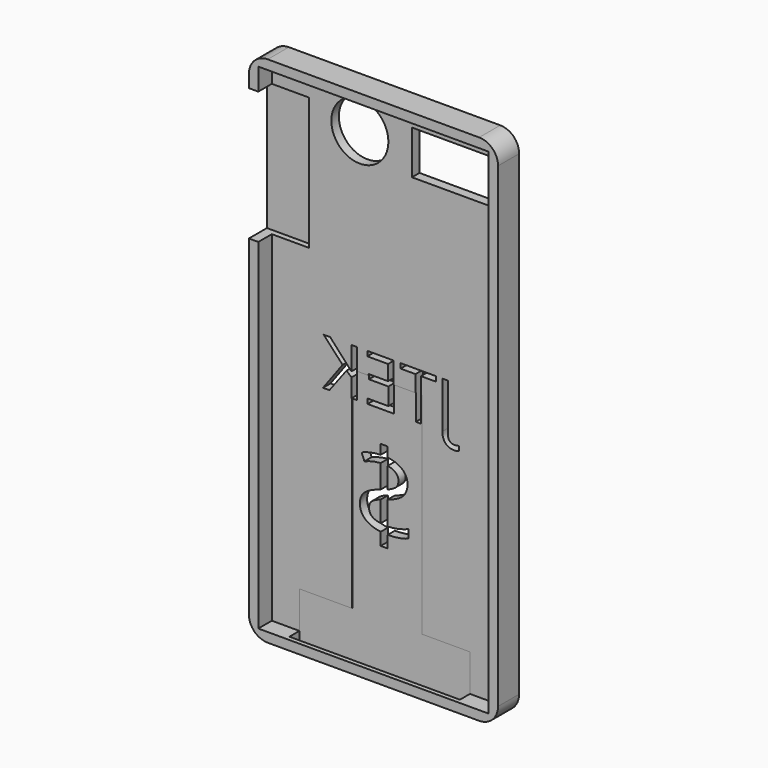
from build123d import *

# Parameters (mm, degrees)
F0_W          = 67.1
F0_H          = 138.3
F1_DEPTH      = 3.55
F2_T          = -2.54
F3_R          = 5.08
F4_R          = 5.08
F5_R          = 5.08
F6_R          = 5.08
F7_W          = 21.1026063189
F7_H          = 11.7926336825
F8_DEPTH      = 12.5
F11_W         = 18.811494112
F11_H         = 2.224416472
F12_DEPTH     = 91.3
F13_W         = 6.076481403
F13_H         = 22.8435061872
F14_DEPTH     = 12.5
F15_R         = 7.6799420763
F16_DEPTH     = 25
F18_DEPTH     = 12.5
F19_W         = 6.076481403
F19_H         = 12.7864610404
F20_DEPTH     = 12.5
F21_R         = 12.4287967825
F22_DEPTH     = 25
F23_DEPTH     = 108.6
F24_TEXT_SIZE = 17.723527142
F25_DEPTH     = 12.5
F26_TEXT_SIZE = 29.6242431634
F27_DEPTH     = 25


# Not quite as in the source:
# - a feature of the source that left no trace in its solid (it failed there, or was rolled back) is left out
# - Text() gives the source's letters only with a copy of the font that has no kerning and outlines rounded to 1/6400 em; it was checked with that copy


with BuildPart() as f1:
    # F0 (on Front) → F1 (new body, symmetric)
    with BuildSketch(Plane.XZ):
        Rectangle(F0_W, F0_H)
    extrude(amount=F1_DEPTH, both=True)

    # F2
    f2_openings = [f1.faces().sort_by_distance(p)[0] for p in [
        (0, -3.55, 0),
    ]]
    offset(amount=F2_T, openings=f2_openings)

    # F3
    f3_edges = [f1.edges().sort_by_distance(p)[0] for p in [
        (33.55, 0, 69.15),
    ]]
    fillet(f3_edges, radius=F3_R)

    # F4
    f4_edges = [f1.edges().sort_by_distance(p)[0] for p in [
        (-33.55, 0, 69.15),
    ]]
    fillet(f4_edges, radius=F4_R)

    # F5
    f5_edges = [f1.edges().sort_by_distance(p)[0] for p in [
        (-33.55, 0, -69.15),
    ]]
    fillet(f5_edges, radius=F5_R)

    # F6
    f6_edges = [f1.edges().sort_by_distance(p)[0] for p in [
        (33.55, 0, -69.15),
    ]]
    fillet(f6_edges, radius=F6_R)

    # F7 (on face) → F8 (cut, symmetric)
    with BuildSketch(Plane.XZ.offset(-1.01)):
        with Locations((17.2698632814, 56.677794084)):
            Rectangle(F7_W, F7_H)
    extrude(amount=F8_DEPTH, both=True, mode=Mode.SUBTRACT)

    # F11 (on Top) → F12 (cut)
    with BuildSketch(Plane.XY):
        Rectangle(F11_W, F11_H)
    extrude(amount=-F12_DEPTH, mode=Mode.SUBTRACT)

    # F13 (on face) → F14 (cut, symmetric)
    with BuildSketch(Plane(origin=(-33.55, 0, 0), x_dir=(0, -1, 0), z_dir=(-1, 0, 0))):
        with Locations((0.5117592985, 49.2424760014)):
            Rectangle(F13_W, F13_H)
    extrude(amount=F14_DEPTH, both=True, mode=Mode.SUBTRACT)

    # F15 (on face) → F16 (cut)
    with BuildSketch(Plane.XZ.offset(-1.01)):
        with Locations((-7.3086209595, 57.1251362562)):
            Circle(F15_R)
    extrude(amount=-F16_DEPTH, mode=Mode.SUBTRACT)

    # F17 (on face) → F18 (cut, symmetric)
    with BuildSketch(Plane(origin=(0, 0, -69.15), x_dir=(1, 0, 0), z_dir=(0, 0, -1))):
        Polygon((22.3355982453, 2.3663339671), (-23.5800333321, 2.3663339671), (-23.5800333321, -1.112208236), (-9.405747056, -1.112208236), (-9.405747056, 1.112208236), (9.405747056, 1.112208236), (9.405747056, -1.112208236), (22.3355982453, -1.112208236), align=None)
    extrude(amount=F18_DEPTH, both=True, mode=Mode.SUBTRACT)

    # F19 (on face) → F20 (cut, symmetric)
    with BuildSketch(Plane(origin=(-33.55, 0, 0), x_dir=(0, -1, 0), z_dir=(-1, 0, 0))):
        with Locations((0.5117592985, 31.4274923876)):
            Rectangle(F19_W, F19_H)
    extrude(amount=F20_DEPTH, both=True, mode=Mode.SUBTRACT)

    # F24 (on face) → F25 (cut, symmetric)
    with BuildSketch(Plane(origin=(0, 3.55, 0), x_dir=(-1, 0, 0), z_dir=(0, 1, 0))):
        with Locations((-18.0315598845, -6.9183185697)):
            Text('JTEK', F24_TEXT_SIZE, font='Open Sans', text_align=(TextAlign.LEFT, TextAlign.BOTTOM))
    extrude(amount=F25_DEPTH, both=True, mode=Mode.SUBTRACT)

    # F26 (on face) → F27 (cut)
    with BuildSketch(Plane(origin=(0, 3.55, 0), x_dir=(-1, 0, 0), z_dir=(0, 1, 0))):
        with Locations((-7.6080858707, -37.6916863024)):
            Text('$', F26_TEXT_SIZE, font='Open Sans', text_align=(TextAlign.LEFT, TextAlign.BOTTOM))
    extrude(amount=-F27_DEPTH, mode=Mode.SUBTRACT)


with BuildPart() as f22:
    # F21 (on face) → F22 (new body)
    with BuildSketch(Plane(origin=(0, 3.55, 0), x_dir=(-1, 0, 0), z_dir=(0, 1, 0))):
        with Locations((-5.5705006234, -36.2981520593)):
            Circle(F21_R)
    extrude(amount=F22_DEPTH)

    # F23 (cut, symmetric): a face of the model
    f23_faces = [f22.faces().sort_by_distance(p)[0] for p in [
        (5.5705006234, 28.55, -36.2981520593),
    ]]
    extrude(f23_faces, amount=F23_DEPTH, both=True, mode=Mode.SUBTRACT)


solid = f1.part
